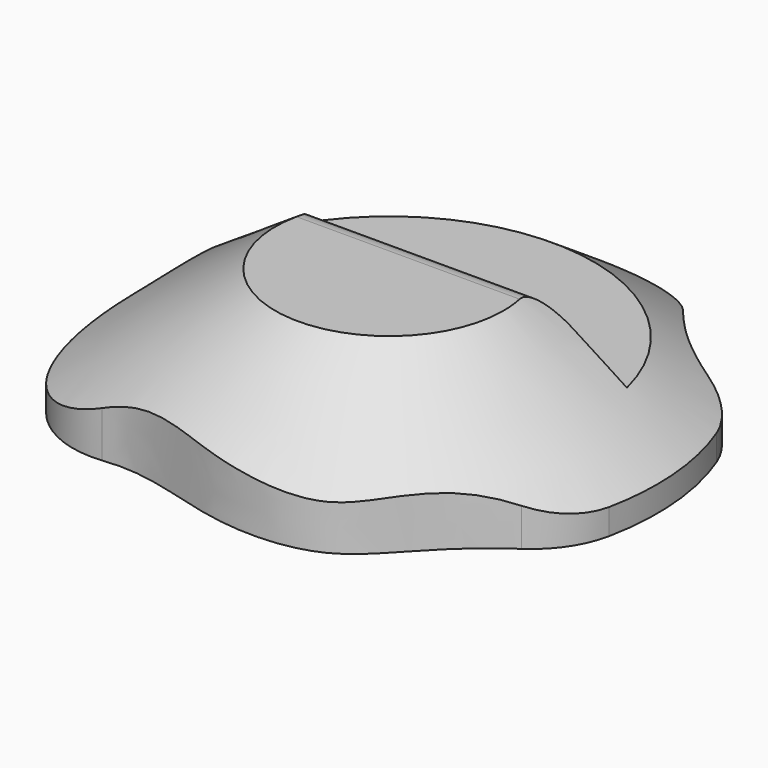
from build123d import *

# Parameters (mm, degrees)
F0_R          = 26.5230501381
F1_DEPTH      = 12.7
F2_SIZE2      = 10.16
F2_SIZE       = 15.24
F4_W          = 22.5503575057
F4_H          = 12.9768685438
F5_DEPTH      = 72.898
F6_R          = 2.54
F9_DEPTH      = 13.97
F10_R         = 9.2046108509
F11_DEPTH     = 12.446
F12_T1_DEPTH  = 42.6936272055
F12_T3_DEPTH  = 20.1925030817
F12_T5_DEPTH  = 28.3416358411
F12_T7_DEPTH  = 27.2837343834
F12_T9_DEPTH  = 34.6744237305
F12_T11_DEPTH = 25.9767712333
F12_T13_DEPTH = 47.1089861743
F13_SCALE     = 1.2


# Not quite as in the source:
# - a fillet or chamfer that OpenCascade refuses, or shapes differently, is made with other operations: its cross-section is extruded or revolved along the edge and cut away or added


with BuildPart() as f1:
    # F0 (on Top) → F1 (new body)
    with BuildSketch(Plane.XY):
        with Locations((-30.8415237814, 0)):
            Circle(F0_R)
    extrude(amount=F1_DEPTH)

    # F2
    f2_edges = [f1.edges().sort_by_distance(p)[0] for p in [
        (-57.364574, 0, 12.7),
    ]]
    f2_side = f1.faces().sort_by_distance((-30.841524, 0, 12.7))[0]
    chamfer(f2_edges, length=F2_SIZE, length2=F2_SIZE2, reference=f2_side)

    # F4 (on Right) → F5 (cut)
    with BuildSketch(Plane.YZ):
        with Locations((16.1333801225, 13.2286406588)):
            Rectangle(F4_W, F4_H)
    extrude(amount=-F5_DEPTH, mode=Mode.SUBTRACT)

    # F6
    f6_edges = [f1.edges().sort_by_distance(p)[0] for p in [
        (-30.841524, 4.858201, 12.7),
    ]]
    fillet(f6_edges, radius=F6_R)

    # F8 (on Top) → F9 (cut)
    with BuildSketch(Plane.XY):
        with BuildLine():
            add(Edge.make_bspline(
                [(-55.3713850677, 22.9514930397), (-49.78992436, 18.7102913876), (-40.1413659504, 13.1276116135), (-26.057679824, 35.9571873343), (-15.9947189321, 13.1009864119), (4.8109050938, 12.5958076193), (2.8427049911, 53.374611772), (-81.2467530092, 45.4711212768), (-61.4883008278, 27.5995725634), (-55.3713850677, 22.9514930397)],
                knots=[0, 0, 0, 0, 0.1200214926, 0.2444612, 0.3709842799, 0.4839706118, 0.6355466034, 0.8684642967, 1, 1, 1, 1], degree=3))
        make_face()
        with BuildLine():
            add(Edge.make_bspline(
                [(-51.0003603995, -23.0153966695), (-48.1362609461, -20.6798155927), (-40.7003687035, -18.5550660634), (-30.9746254877, -22.7368211073), (-19.133870658, -22.4424322322), (-13.8967054425, -14.1578655221), (2.7182633946, -3.071907799), (2.9022796426, -41.6881399026), (-59.8070800541, -35.1672051718), (-53.4295629739, -24.9963333153), (-51.0003603995, -23.0153966695)],
                knots=[0, 0, 0, 0, 0.1057878637, 0.2117160634, 0.3164559902, 0.4209969049, 0.5358573163, 0.6850300725, 0.9102754094, 1, 1, 1, 1], degree=3))
        make_face()
    extrude(amount=F9_DEPTH, mode=Mode.SUBTRACT)

    # F10 (on Top) → F11 (cut)
    with BuildSketch(Plane.XY):
        with Locations((-59.7444288433, 0)):
            Circle(F10_R)
    extrude(amount=F11_DEPTH, mode=Mode.SUBTRACT)

    # F12: fillet of radius 9.4234 on 8 edges, made by hand

    # F12_s2 → F12_t1 (cut)
    with BuildSketch(Plane.XY.offset(-20.0768133028)):
        with BuildLine():
            ThreePointArc((-44.8287256922, 17.4618663374), (-50.267472068, 16.450270163), (-54.201876195, 12.5613431742))
            Line((-54.201876195, 12.5613431742), (-55.0320219668, 13.0077296729))
            ThreePointArc((-55.0320219668, 13.0077296729), (-52.7836593667, 16.519744157), (-50.0298041231, 19.6511872055))
            Line((-50.0298041231, 19.6511872055), (-48.9381460051, 19.8139284253))
            ThreePointArc((-48.9381460051, 19.8139284253), (-46.8608710208, 18.9051311498), (-44.7215564137, 18.3983051525))
            Line((-44.7215564137, 18.3983051525), (-44.8287256922, 17.4618663374))
        make_face()
    extrude(amount=F12_T1_DEPTH, mode=Mode.SUBTRACT)

    # F12_s4 → F12_t3 (cut)
    with BuildSketch(Plane.XY.offset(-8.8262512408)):
        with BuildLine():
            ThreePointArc((-19.8798828029, 22.6453151082), (-22.2566439848, 24.731584944), (-25.1896863188, 25.9142844879))
            Line((-25.1896863188, 25.9142844879), (-24.9888335289, 26.8352161973))
            ThreePointArc((-24.9888335289, 26.8352161973), (-23.2159215366, 26.3858111356), (-21.4767132582, 25.8197823915))
            Line((-21.4767132582, 25.8197823915), (-21.0941936793, 25.5605612647))
            ThreePointArc((-21.0941936793, 25.5605612647), (-20.1017662371, 24.4028509916), (-19.1480496615, 23.2393498795))
            Line((-19.1480496615, 23.2393498795), (-19.8798828029, 22.6453151082))
        make_face()
    extrude(amount=F12_T3_DEPTH, mode=Mode.SUBTRACT)

    # F12_s6 → F12_t5 (cut)
    with BuildSketch(Plane.XY.offset(-12.9008176205)):
        with BuildLine():
            ThreePointArc((-25.3871072246, 25.9565549958), (-29.9431154078, 25.7872516977), (-33.8867145439, 23.49947985))
            Line((-33.8867145439, 23.49947985), (-34.5428383529, 24.1762062375))
            ThreePointArc((-34.5428383529, 24.1762062375), (-32.8806872828, 25.7527274974), (-31.0877935592, 27.2707519289))
            Line((-31.0877935592, 27.2707519289), (-30.5049130386, 27.4635673591))
            ThreePointArc((-30.5049130386, 27.4635673591), (-27.8348524929, 27.3005634858), (-25.1932703017, 26.8789888979))
            Line((-25.1932703017, 26.8789888979), (-25.3871072246, 25.9565549958))
        make_face()
    extrude(amount=F12_T5_DEPTH, mode=Mode.SUBTRACT)

    # F12_s8 → F12_t7 (cut)
    with BuildSketch(Plane.XY.offset(-12.3718668917)):
        with BuildLine():
            ThreePointArc((-11.1528795968, 14.7745936831), (-8.0771007987, 12.6445190663), (-6.0722794793, 9.4856704523))
            Line((-6.0722794793, 9.4856704523), (-5.1920397604, 9.8227684998))
            ThreePointArc((-5.1920397604, 9.8227684998), (-6.2206226761, 12.1725949429), (-7.4635970901, 14.416427522))
            Line((-7.4635970901, 14.416427522), (-8.1134854062, 14.8518537835))
            ThreePointArc((-8.1134854062, 14.8518537835), (-9.4672167518, 15.1637501963), (-10.7806998896, 15.6405840537))
            Line((-10.7806998896, 15.6405840537), (-11.1528795968, 14.7745936831))
        make_face()
    extrude(amount=F12_T7_DEPTH, mode=Mode.SUBTRACT)

    # F12_s10 → F12_t9 (cut)
    with BuildSketch(Plane.XY.offset(-16.0672115653)):
        with BuildLine():
            ThreePointArc((-51.785250315, -16.2743272093), (-48.0161691892, -19.1711869731), (-43.3126579557, -19.8602088168))
            Line((-43.3126579557, -19.8602088168), (-43.2096886841, -20.7971476545))
            ThreePointArc((-43.2096886841, -20.7971476545), (-45.0909873153, -21.1305134729), (-46.9093149737, -21.7103687863))
            Line((-46.9093149737, -21.7103687863), (-47.839075605, -21.5741528428))
            ThreePointArc((-47.839075605, -21.5741528428), (-50.3277123461, -19.3558594256), (-52.5295402792, -16.8526778862))
            Line((-52.5295402792, -16.8526778862), (-51.785250315, -16.2743272093))
        make_face()
    extrude(amount=F12_T9_DEPTH, mode=Mode.SUBTRACT)

    # F12_s12 → F12_t11 (cut)
    with BuildSketch(Plane.XY.offset(-11.7183853166)):
        with BuildLine():
            ThreePointArc((-8.8600313718, -11.2068288558), (-6.249192378, -8.6076622776), (-4.8340580996, -5.2062593132))
            Line((-4.8340580996, -5.2062593132), (-3.9098149535, -5.391277321))
            ThreePointArc((-3.9098149535, -5.391277321), (-4.4919315636, -7.7498276648), (-5.279808144, -10.0478620887))
            Line((-5.279808144, -10.0478620887), (-5.7809831263, -10.5673442739))
            ThreePointArc((-5.7809831263, -10.5673442739), (-7.0796673825, -11.2179342277), (-8.3383855529, -11.9919038178))
            Line((-8.3383855529, -11.9919038178), (-8.8600313718, -11.2068288558))
        make_face()
    extrude(amount=F12_T11_DEPTH, mode=Mode.SUBTRACT)

    # F12_s14 → F12_t13 (cut)
    with BuildSketch(Plane.XY.offset(-22.2844930871)):
        with BuildLine():
            ThreePointArc((-51.7913199374, 16.2665130944), (-53.7673063587, 10.7799856189), (-52.1369049751, 5.1810305908))
            Line((-52.1369049751, 5.1810305908), (-52.9159013196, 4.6505026608))
            ThreePointArc((-52.9159013196, 4.6505026608), (-54.4464619427, 6.3398832318), (-56.3805976711, 7.5463376891))
            Line((-56.3805976711, 7.5463376891), (-56.8907643621, 8.7059282809))
            ThreePointArc((-56.8907643621, 8.7059282809), (-55.0574218125, 12.9594137449), (-52.5357577781, 16.8445334147))
            Line((-52.5357577781, 16.8445334147), (-51.7913199374, 16.2665130944))
        make_face()
        with BuildLine():
            ThreePointArc((-52.1369049751, -5.1810305908), (-53.7673063587, -10.7799856189), (-51.7913199374, -16.2665130944))
            Line((-51.7913199374, -16.2665130944), (-52.5357577781, -16.8445334147))
            ThreePointArc((-52.5357577781, -16.8445334147), (-55.0574218125, -12.9594137449), (-56.8907643621, -8.7059282809))
            Line((-56.8907643621, -8.7059282809), (-56.3805976711, -7.5463376891))
            ThreePointArc((-56.3805976711, -7.5463376891), (-54.4464619427, -6.3398832318), (-52.9159013196, -4.6505026608))
            Line((-52.9159013196, -4.6505026608), (-52.1369049751, -5.1810305908))
        make_face()
    extrude(amount=F12_T13_DEPTH, mode=Mode.SUBTRACT)


with BuildPart() as f13_1:
    # F13: copy of F1
    add(f1.part.scale(F13_SCALE).moved(Location((6.1397526413, 0.5236500409, -2.54))))


with BuildPart() as f13_1_1:
    # F14: moved
    add(f13_1.part.moved(Location((0, 0, 2.6416))))

    # F15: cut F1
    add(f1.part, mode=Mode.SUBTRACT)


solid = f13_1_1.part
